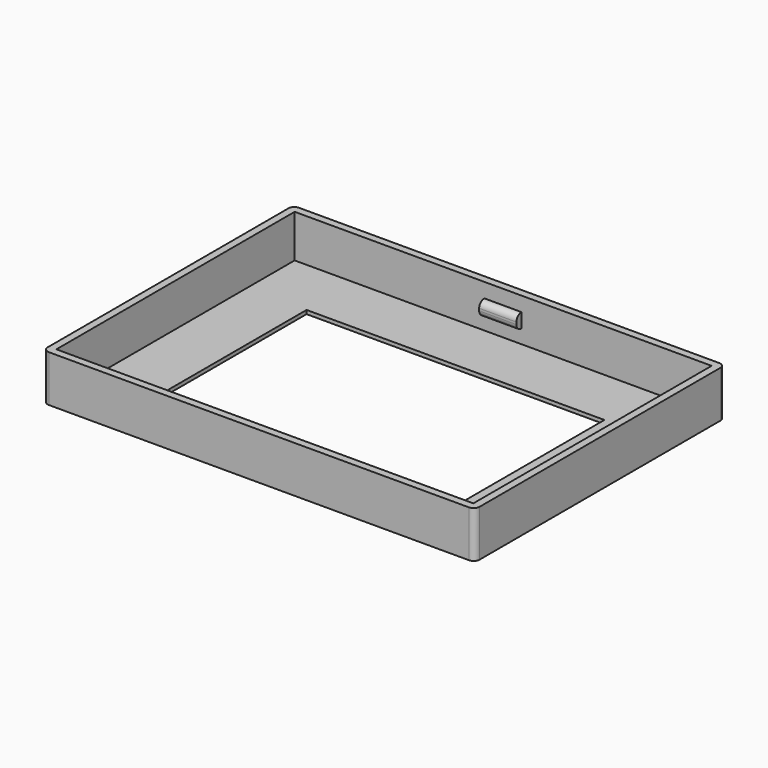
from build123d import *

# Parameters (mm, degrees)
F0_W     = 56
F0_H     = 40
F0_W_2   = 40
F0_H_2   = 24
F1_DEPTH = 0.5
F0_W_3   = 58
F0_H_3   = 42
F2_DEPTH = 6.25
F3_W     = 5
F3_H     = 1.9
F4_DEPTH = 0.9
F5_R     = 0.8


# Not quite as in the source:
# - two fillets or chamfers of one size are made in one step
# - a pattern or mirror of a feature is missing from the dataset's text; its kind, count and spacing are read off the source's solid


with BuildPart() as f1:
    # F0 (on Top) → F1 (new body)
    with BuildSketch(Plane.XY):
        Rectangle(F0_W, F0_H)
        Rectangle(F0_W_2, F0_H_2, mode=Mode.SUBTRACT)
    extrude(amount=F1_DEPTH)

    # F0 (on Top) → F2 (join)
    with BuildSketch(Plane.XY):
        Rectangle(F0_W_3, F0_H_3)
        Rectangle(F0_W, F0_H, mode=Mode.SUBTRACT)
    extrude(amount=F2_DEPTH)

    # F3 (on face) → F4 (join)
    with BuildSketch(Plane(origin=(0, -20, 0), x_dir=(-1, 0, 0), z_dir=(0, 1, 0))):
        with Locations((0, 3.35)):
            Rectangle(F3_W, F3_H)
    f4 = extrude(amount=F4_DEPTH)

    # F4_copies: F4 across plane
    add(f4.mirror(Plane.ZX))

    # F5
    f5_edges = [f1.edges().sort_by_distance(p)[0] for p in [
        (0, -19.1, 4.3),
        (0, -19.1, 2.4),
        (29, 21, 3.125),
        (-29, 21, 3.125),
        (-29, -21, 3.125),
        (29, -21, 3.125),
        (0, 19.1, 4.3),
        (0, 19.1, 2.4),
    ]]
    fillet(f5_edges, radius=F5_R)


solid = f1.part
